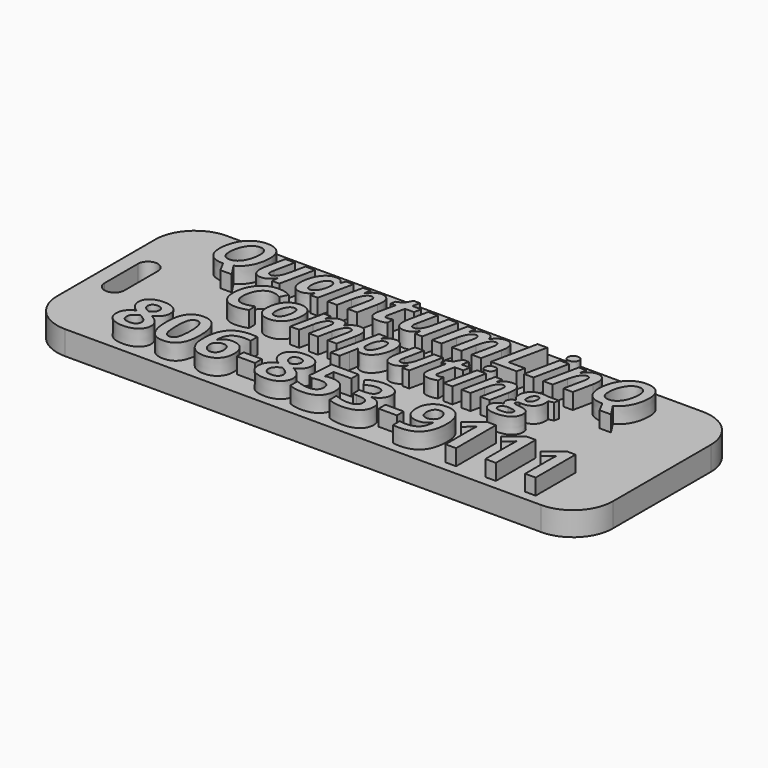
from build123d import *

# Parameters (mm, degrees)
F0_W           = 69.85
F0_H           = 25.4
F1_DEPTH       = 3
F3_R           = 5
F2_TEXT_SIZE   = 8.1216017457
F2_TEXT_SIZE_2 = 7.6601472554
F2_TEXT_SIZE_3 = 8.7680812511
F4_DEPTH       = 2
F6_DEPTH       = 25


# Not quite as in the source:
# - Text() gives the source's letters only with a copy of the font that has no kerning and outlines rounded to 1/6400 em; it was checked with that copy


with BuildPart() as f1:
    # F0 (on Top) → F1 (new body)
    with BuildSketch(Plane.XY):
        Rectangle(F0_W, F0_H)
    extrude(amount=F1_DEPTH)

    # F3
    f3_edges = [f1.edges().sort_by_distance(p)[0] for p in [
        (-34.925, -12.7, 1.5),
        (-34.925, 12.7, 1.5),
        (34.925, -12.7, 1.5),
        (34.925, 12.7, 1.5),
    ]]
    fillet(f3_edges, radius=F3_R)

    # F2 (on face) → F4 (join)
    with BuildSketch(Plane.XY.offset(3)):
        with Locations((-26.914473623, 4.9964431673)):
            Text('QuantumLinQ', F2_TEXT_SIZE, font='Open Sans', font_style=FontStyle.BOLDITALIC, text_align=(TextAlign.LEFT, TextAlign.BOTTOM))
        with Locations((-19.9372749776, -1.4491558541)):
            Text('Computing', F2_TEXT_SIZE_2, font='Open Sans', font_style=FontStyle.BOLDITALIC, text_align=(TextAlign.LEFT, TextAlign.BOTTOM))
        with Locations((-26.0506290942, -11.4840036258)):
            Text('806-853-9111', F2_TEXT_SIZE_3, font='Open Sans', font_style=FontStyle.BOLD, text_align=(TextAlign.LEFT, TextAlign.BOTTOM))
    extrude(amount=F4_DEPTH)

    # F5 (on face) → F6 (cut)
    with BuildSketch(Plane.XY.offset(3)):
        with BuildLine():
            ThreePointArc((-33.0246624351, -2.625), (-31.7746624351, -3.875), (-30.5246624351, -2.625))
            Line((-30.5246624351, -2.625), (-30.5246624351, 2.625))
            ThreePointArc((-30.5246624351, 2.625), (-31.7746624351, 3.875), (-33.0246624351, 2.625))
            Line((-33.0246624351, 2.625), (-33.0246624351, -2.625))
        make_face()
    extrude(amount=-F6_DEPTH, mode=Mode.SUBTRACT)


solid = f1.part
